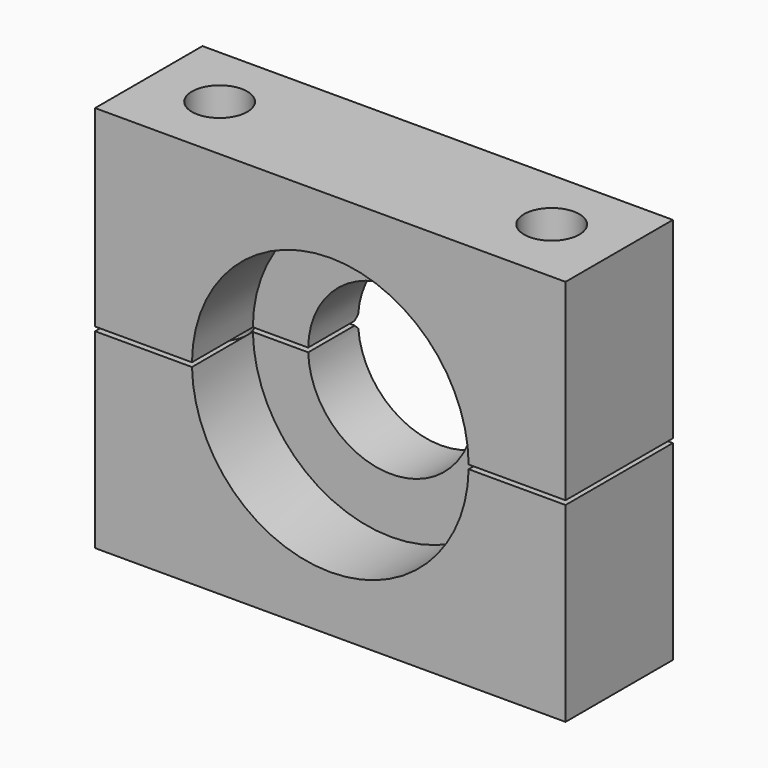
from build123d import *

# Parameters (mm, degrees)
F0_W             = 34
F0_H             = 13.9
F1_DEPTH         = 10
F0_H_2           = 13.8
F2_D             = 12
F2_CBORE_D       = 20
F2_CBORE_DEPTH   = 5.5
F2_2_D           = 12
F2_2_CBORE_D     = 20
F2_2_CBORE_DEPTH = 5.5
F4_D             = 4
F4_CBORE_D       = 8
F4_CBORE_DEPTH   = 4
F4_2_D           = 4
F4_2_CBORE_D     = 8
F4_2_CBORE_DEPTH = 4
F5_SIZE          = 0.3
F5_2_SIZE        = 0.3


# Not quite as in the source:
# - a feature names something its author has since deleted; it is built from what else it names


with BuildPart() as f1:
    # F0 (on Front) → F1 (new body)
    with BuildSketch(Plane.XZ):
        with Locations((0, 7.05)):
            Rectangle(F0_W, F0_H)
    extrude(amount=-F1_DEPTH)

    # F2 (through all)
    with Locations(Plane.XZ):
        with Locations((0, 0)):
            CounterBoreHole(F2_D / 2, F2_CBORE_D / 2, F2_CBORE_DEPTH)

    # F4 (through all)
    with Locations(Plane(origin=(0, 0, -14), x_dir=(1, 0, 0), z_dir=(0, 0, -1))):
        with Locations((-12, -5), (12, -5)):
            CounterBoreHole(F4_D / 2, F4_CBORE_D / 2, F4_CBORE_DEPTH)

    # F5
    f5_edges = [f1.edges().sort_by_distance(p)[0] for p in [
        (0, 10, 14),
        (-17, 10, 7.05),
        (17, 10, 7.05),
        (11.499583, 10, 0.1),
        (-11.499583, 10, 0.1),
    ]]
    chamfer(f5_edges, length=F5_SIZE)


with BuildPart() as f1b:
    # F0 (on Front) → F1, piece 2 (new body)
    with BuildSketch(Plane.XZ):
        with Locations((0, -7.1)):
            Rectangle(F0_W, F0_H_2)
    extrude(amount=-F1_DEPTH)

    # F2#2 (through all)
    with Locations(Plane.XZ):
        with Locations((0, 0)):
            CounterBoreHole(F2_2_D / 2, F2_2_CBORE_D / 2, F2_2_CBORE_DEPTH)

    # F4#2 (through all)
    with Locations(Plane(origin=(0, 0, -14), x_dir=(1, 0, 0), z_dir=(0, 0, -1))):
        with Locations((-12, -5), (12, -5)):
            CounterBoreHole(F4_2_D / 2, F4_2_CBORE_D / 2, F4_2_CBORE_DEPTH)

    # F5#2
    f5_2_edges = [f1b.edges().sort_by_distance(p)[0] for p in [
        (-17, 10, -7.1),
        (17, 10, -7.1),
        (0, 10, -14),
        (11.498333, 10, -0.2),
        (-11.498333, 10, -0.2),
    ]]
    chamfer(f5_2_edges, length=F5_2_SIZE)


solid = Compound([f1.part, f1b.part])
